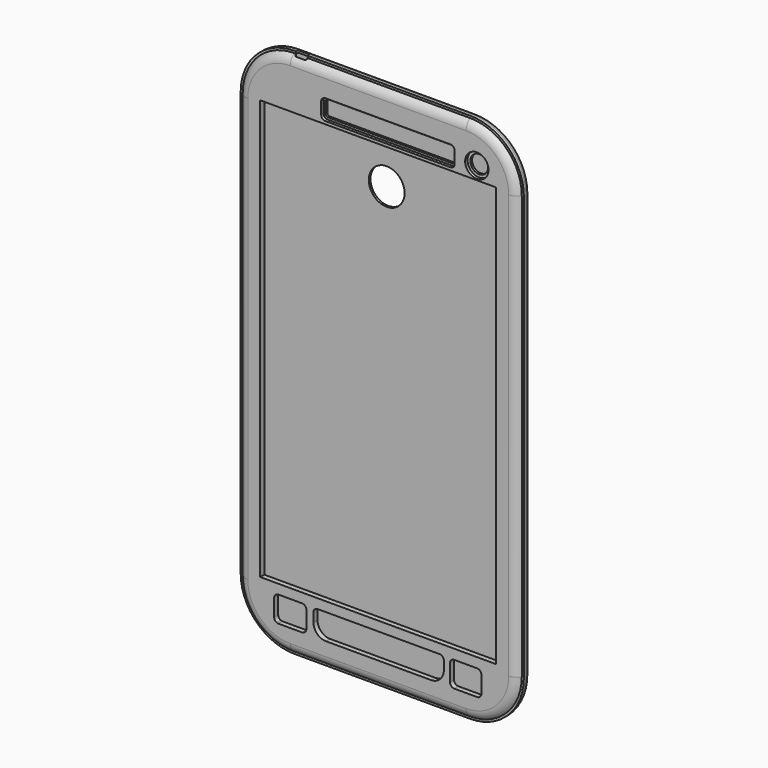
from build123d import *

# Parameters (mm, degrees)
F1_DEPTH       = 1.8
F2_T           = -0.5
F3_TEXT_SIZE   = 14.8850909021
F4_DEPTH       = 0.4
F6_DEPTH       = 1.2
F7_T1_DEPTH    = 100.1693180323
F7_T3_DEPTH    = 41.579196465
F7_T6_ANGLE    = 90
F7_T8_ANGLE    = 90
F7_T10_ANGLE   = 90
F7_T12_ANGLE   = 90
F8_R           = 1.2
F10_W          = 55.8126681519
F10_H          = 99.2564819753
F11_DEPTH      = 5.0007207319
F13_DEPTH      = 25
F14_R          = 2.7675954625
F14_R_2        = 2.0923613447
F15_DEPTH      = 0.6937347353
F16_DEPTH      = 3
F19_DEPTH      = 25
F20_R          = 4.2318258576
F21_DEPTH      = 25
F23_DEPTH      = 10
F23_DEPTH_BACK = 25


# Not quite as in the source:
# - a fillet or chamfer that OpenCascade refuses, or shapes differently, is made with other operations: its cross-section is extruded or revolved along the edge and cut away or added
# - Text() gives the source's letters only with a copy of the font that has no kerning and outlines rounded to 1/6400 em; it was checked with that copy


with BuildPart() as f1:
    # F0 (on Front) → F1 (new body)
    with BuildSketch(Plane.XZ):
        with BuildLine():
            Line((25.4936250091, 55.1304519176), (-16.085571456, 55.1304519176))
            ThreePointArc((-16.085571456, 55.1304519176), (-25.065827577, 51.4107080387), (-28.785571456, 42.4304519176))
            Line((-28.785571456, 42.4304519176), (-28.785571456, -57.7388661146))
            ThreePointArc((-28.785571456, -57.7388661146), (-25.065827577, -66.7191222357), (-16.085571456, -70.4388661146))
            Line((-16.085571456, -70.4388661146), (25.4936250091, -70.4388661146))
            ThreePointArc((25.4936250091, -70.4388661146), (34.4738811301, -66.7191222357), (38.1936250091, -57.7388661146))
            Line((38.1936250091, -57.7388661146), (38.1936250091, 42.4304519176))
            ThreePointArc((38.1936250091, 42.4304519176), (34.4738811301, 51.4107080387), (25.4936250091, 55.1304519176))
        make_face()
    extrude(amount=F1_DEPTH)

    # F2
    f2_openings = [f1.faces().sort_by_distance(p)[0] for p in [
        (4.704027, -1.8, -7.654207),
    ]]
    offset(amount=F2_T, openings=f2_openings)

    # F3 (on face) → F4 (join)
    with BuildSketch(Plane(origin=(0, 0, 0), x_dir=(-1, 0, 0), z_dir=(0, 1, 0))):
        with Locations((-21.8003056943, 37.4392606318)):
            Text('Asus', F3_TEXT_SIZE, font='Open Sans', font_style=FontStyle.BOLD, text_align=(TextAlign.LEFT, TextAlign.BOTTOM))
        with Locations((-17.9325078553, 17.195537005)):
            Text('ZEN', F3_TEXT_SIZE, font='Open Sans', font_style=FontStyle.BOLD, text_align=(TextAlign.LEFT, TextAlign.BOTTOM))
        with Locations((-6.329114338, -3.0481866218)):
            Text('5', F3_TEXT_SIZE, font='Open Sans', font_style=FontStyle.BOLD, text_align=(TextAlign.LEFT, TextAlign.BOTTOM))
    extrude(amount=F4_DEPTH)

    # F8
    f8_edges = [f1.edges().sort_by_distance(p)[0] for p in [
        (-25.065828, 0, -66.719122),
        (4.704027, 0, -70.438866),
        (34.473881, 0, -66.719122),
        (38.193625, 0, -7.654207),
        (-28.785571, 0, -7.654207),
        (-25.065828, 0, 51.410708),
        (4.704027, 0, 55.130452),
        (34.473881, 0, 51.410708),
    ]]
    fillet(f8_edges, radius=F8_R)

    # F18 (on face) → F19 (cut)
    with BuildSketch(Plane(origin=(0, 0, -70.4388661146), x_dir=(1, 0, 0), z_dir=(0, 0, -1))):
        with BuildLine():
            Line((6.5061416602, 1.2), (2.9019118929, 1.2))
            Line((2.9019118929, 1.2), (2.9019118929, 0.8308712449))
            ThreePointArc((2.9019118929, 0.8308712449), (2.9897798586, 0.6187392105), (3.2019118929, 0.5308712449))
            Line((3.2019118929, 0.5308712449), (4.7040267766, 0.5308712449))
            Line((4.7040267766, 0.5308712449), (6.2061416602, 0.5308712449))
            ThreePointArc((6.2061416602, 0.5308712449), (6.4182736945, 0.6187392105), (6.5061416602, 0.8308712449))
            Line((6.5061416602, 0.8308712449), (6.5061416602, 1.2))
        make_face()
        Polygon((6.5061416602, 1.6659845887), (4.7040267766, 1.6659845887), (2.9019118929, 1.6659845887), (2.9019118929, 1.2), (6.5061416602, 1.2), align=None)
    extrude(amount=-F19_DEPTH, mode=Mode.SUBTRACT)

    # F20 (on face) → F21 (cut)
    with BuildSketch(Plane(origin=(0, 0, 0), x_dir=(-1, 0, 0), z_dir=(0, 1, 0))):
        with Locations((-4.7040267766, 33.0976899713)):
            Circle(F20_R)
    extrude(amount=-F21_DEPTH, mode=Mode.SUBTRACT)


with BuildPart() as f6:
    # F5 (on face) → F6 (new body)
    with BuildSketch(Plane.XZ.offset(1.8)):
        with BuildLine():
            ThreePointArc((37.6936250091, 42.4304519176), (34.1203277395, 51.0571546481), (25.4936250091, 54.6304519176))
            Line((25.4936250091, 54.6304519176), (-16.085571456, 54.6304519176))
            ThreePointArc((-16.085571456, 54.6304519176), (-24.7122741864, 51.0571546481), (-28.285571456, 42.4304519176))
            Line((-28.285571456, 42.4304519176), (-28.285571456, -57.7388661146))
            ThreePointArc((-28.285571456, -57.7388661146), (-24.7122741864, -66.3655688451), (-16.085571456, -69.9388661146))
            Line((-16.085571456, -69.9388661146), (25.4936250091, -69.9388661146))
            ThreePointArc((25.4936250091, -69.9388661146), (34.1203277395, -66.3655688451), (37.6936250091, -57.7388661146))
            Line((37.6936250091, -57.7388661146), (37.6936250091, 42.4304519176))
        make_face()
    extrude(amount=F6_DEPTH)

    # F7: fillet of radius 2.5 on 2 edges, made by hand

    # F7_s2 → F7_t1 (cut)
    with BuildSketch(Plane.XY.offset(-57.7388661146)):
        with BuildLine():
            ThreePointArc((37.6936250091, -1.8), (36.78295423, -2.6794494718), (35.5582093587, -3))
            Line((35.5582093587, -3), (35.5582093587, -3.05))
            Line((35.5582093587, -3.05), (37.6936250091, -3.05))
            Line((37.6936250091, -3.05), (37.7436250091, -3))
            ThreePointArc((37.7436250091, -3), (37.7436250091, -2.4), (37.7363333221, -1.826))
            Line((37.7363333221, -1.826), (37.6936250091, -1.8))
        make_face()
        with BuildLine():
            ThreePointArc((-28.285571456, -1.8), (-27.3749006769, -2.6794494718), (-26.1501558055, -3))
            Line((-26.1501558055, -3), (-26.1501558055, -3.05))
            Line((-26.1501558055, -3.05), (-28.285571456, -3.05))
            Line((-28.285571456, -3.05), (-28.335571456, -3))
            ThreePointArc((-28.335571456, -3), (-28.335571456, -2.4), (-28.328279769, -1.826))
            Line((-28.328279769, -1.826), (-28.285571456, -1.8))
        make_face()
    extrude(amount=F7_T1_DEPTH, mode=Mode.SUBTRACT)

    # F7_s4 → F7_t3 (cut)
    with BuildSketch(Plane.YZ.offset(-16.085571456)):
        with BuildLine():
            ThreePointArc((-1.8, 54.6304519176), (-2.6794494718, 53.7197811386), (-3, 52.4950362672))
            Line((-3, 52.4950362672), (-3.05, 52.4950362672))
            Line((-3.05, 52.4950362672), (-3.05, 54.6304519176))
            Line((-3.05, 54.6304519176), (-3, 54.6804519176))
            ThreePointArc((-3, 54.6804519176), (-2.4, 54.6804519176), (-1.826, 54.6731602307))
            Line((-1.826, 54.6731602307), (-1.8, 54.6304519176))
        make_face()
        with BuildLine():
            ThreePointArc((-1.8, -69.9388661146), (-2.6794494718, -69.0281953356), (-3, -67.8034504642))
            Line((-3, -67.8034504642), (-3.05, -67.8034504642))
            Line((-3.05, -67.8034504642), (-3.05, -69.9388661146))
            Line((-3.05, -69.9388661146), (-3, -69.9888661146))
            ThreePointArc((-3, -69.9888661146), (-2.4, -69.9888661146), (-1.826, -69.9815744276))
            Line((-1.826, -69.9815744276), (-1.8, -69.9388661146))
        make_face()
    extrude(amount=F7_T3_DEPTH, mode=Mode.SUBTRACT)

    # F7_s5 → F7_t6 (revolve, cut)
    with BuildSketch(Plane.YZ.offset(25.4936250091)):
        with BuildLine():
            ThreePointArc((-1.8, -69.9388661146), (-2.6794494718, -69.0281953356), (-3, -67.8034504642))
            Line((-3, -67.8034504642), (-3.05, -67.8034504642))
            Line((-3.05, -67.8034504642), (-3.05, -69.9388661146))
            Line((-3.05, -69.9388661146), (-3, -69.9888661146))
            ThreePointArc((-3, -69.9888661146), (-2.4, -69.9888661146), (-1.826, -69.9815744276))
            Line((-1.826, -69.9815744276), (-1.8, -69.9388661146))
        make_face()
    revolve(axis=Axis((25.4936250091, -3, -57.7388661146), (0, -1, 0)), revolution_arc=F7_T6_ANGLE, mode=Mode.SUBTRACT)

    # F7_s7 → F7_t8 (revolve, cut)
    with BuildSketch(Plane.XY.offset(42.4304519176)):
        with BuildLine():
            ThreePointArc((37.6936250091, -1.8), (36.78295423, -2.6794494718), (35.5582093587, -3))
            Line((35.5582093587, -3), (35.5582093587, -3.05))
            Line((35.5582093587, -3.05), (37.6936250091, -3.05))
            Line((37.6936250091, -3.05), (37.7436250091, -3))
            ThreePointArc((37.7436250091, -3), (37.7436250091, -2.4), (37.7363333221, -1.826))
            Line((37.7363333221, -1.826), (37.6936250091, -1.8))
        make_face()
    revolve(axis=Axis((25.4936250091, -3, 42.4304519176), (0, -1, 0)), revolution_arc=F7_T8_ANGLE, mode=Mode.SUBTRACT)

    # F7_s9 → F7_t10 (revolve, cut)
    with BuildSketch(Plane.YZ.offset(-16.085571456)):
        with BuildLine():
            ThreePointArc((-1.8, 54.6304519176), (-2.6794494718, 53.7197811386), (-3, 52.4950362672))
            Line((-3, 52.4950362672), (-3.05, 52.4950362672))
            Line((-3.05, 52.4950362672), (-3.05, 54.6304519176))
            Line((-3.05, 54.6304519176), (-3, 54.6804519176))
            ThreePointArc((-3, 54.6804519176), (-2.4, 54.6804519176), (-1.826, 54.6731602307))
            Line((-1.826, 54.6731602307), (-1.8, 54.6304519176))
        make_face()
    revolve(axis=Axis((-16.085571456, -3, 42.4304519176), (0, -1, 0)), revolution_arc=F7_T10_ANGLE, mode=Mode.SUBTRACT)

    # F7_s11 → F7_t12 (revolve, cut)
    with BuildSketch(Plane.XY.offset(-57.7388661146)):
        with BuildLine():
            ThreePointArc((-28.285571456, -1.8), (-27.3749006769, -2.6794494718), (-26.1501558055, -3))
            Line((-26.1501558055, -3), (-26.1501558055, -3.05))
            Line((-26.1501558055, -3.05), (-28.285571456, -3.05))
            Line((-28.285571456, -3.05), (-28.335571456, -3))
            ThreePointArc((-28.335571456, -3), (-28.335571456, -2.4), (-28.328279769, -1.826))
            Line((-28.328279769, -1.826), (-28.285571456, -1.8))
        make_face()
    revolve(axis=Axis((-16.085571456, -3, -57.7388661146), (0, -1, 0)), revolution_arc=F7_T12_ANGLE, mode=Mode.SUBTRACT)

    # F10 (on face) → F11 (cut)
    with BuildSketch(Plane.XZ.offset(3)):
        with Locations((4.7040267766, -6.6294241697)):
            Rectangle(F10_W, F10_H)
    extrude(amount=-F11_DEPTH, mode=Mode.SUBTRACT)

    # F12 (on face) → F13 (cut)
    with BuildSketch(Plane.XZ.offset(3)):
        with BuildLine():
            ThreePointArc((-12.2817195952, -59.5123114288), (-12.574612814, -58.8052046476), (-13.2817195952, -58.5123114288))
            Line((-13.2817195952, -58.5123114288), (-18.9017766863, -58.5123114288))
            ThreePointArc((-18.9017766863, -58.5123114288), (-19.6088834675, -58.8052046476), (-19.9017766863, -59.5123114288))
            Line((-19.9017766863, -59.5123114288), (-19.9017766863, -63.5656511188))
            ThreePointArc((-19.9017766863, -63.5656511188), (-19.7562864222, -64.0850864961), (-19.3621504639, -64.453376293))
            ThreePointArc((-19.3621504639, -64.453376293), (-19.2387093732, -64.499454064), (-19.1142862352, -64.5428101087))
            ThreePointArc((-19.1142862352, -64.5428101087), (-19.0086434493, -64.559924469), (-18.9017766863, -64.5656511188))
            Line((-18.9017766863, -64.5656511188), (-13.3337015286, -64.5656511188))
            ThreePointArc((-13.3337015286, -64.5656511188), (-12.5898379698, -64.2575327441), (-12.2817195952, -63.5136691853))
            Line((-12.2817195952, -63.5136691853), (-12.2817195952, -59.5123114288))
        make_face()
        with BuildLine():
            Line((29.1073294297, -63.5656511188), (29.1073294297, -59.5850522459))
            ThreePointArc((29.1073294297, -59.5850522459), (28.8144362109, -58.8779454647), (28.1073294297, -58.5850522459))
            Line((28.1073294297, -58.5850522459), (22.6829676867, -58.5850522459))
            ThreePointArc((22.6829676867, -58.5850522459), (21.9758609055, -58.8779454647), (21.6829676867, -59.5850522459))
            Line((21.6829676867, -59.5850522459), (21.6829676867, -63.5656511188))
            ThreePointArc((21.6829676867, -63.5656511188), (21.9758609055, -64.2727578999), (22.6829676867, -64.5656511188))
            Line((22.6829676867, -64.5656511188), (28.1073294297, -64.5656511188))
            ThreePointArc((28.1073294297, -64.5656511188), (28.8144362109, -64.2727578999), (29.1073294297, -63.5656511188))
        make_face()
        with BuildLine():
            ThreePointArc((20.2198089153, -59.5123114288), (19.9269156964, -58.8052046476), (19.2198089153, -58.5123114288))
            Line((19.2198089153, -58.5123114288), (-9.6241041794, -58.5123114288))
            ThreePointArc((-9.6241041794, -58.5123114288), (-10.3312109606, -58.8052046476), (-10.6241041794, -59.5123114288))
            Line((-10.6241041794, -59.5123114288), (-10.6241041794, -61.5703942418))
            ThreePointArc((-10.6241041794, -61.5703942418), (-9.745424523, -63.6917145854), (-7.6241041794, -64.5703942418))
            Line((-7.6241041794, -64.5703942418), (17.2198089153, -64.5703942418))
            ThreePointArc((17.2198089153, -64.5703942418), (19.3411292588, -63.6917145854), (20.2198089153, -61.5703942418))
            Line((20.2198089153, -61.5703942418), (20.2198089153, -59.5123114288))
        make_face()
    extrude(amount=-F13_DEPTH, mode=Mode.SUBTRACT)

    # F14 (on face) → F15 (cut)
    with BuildSketch(Plane.XZ.offset(3)):
        with BuildLine():
            Line((21.8011573888, 48.4449677169), (-7.7840846498, 48.4449677169))
            ThreePointArc((-7.7840846498, 48.4449677169), (-8.4911914309, 48.1520744981), (-8.7840846498, 47.4449677169))
            Line((-8.7840846498, 47.4449677169), (-8.7840846498, 44.6754697382))
            ThreePointArc((-8.7840846498, 44.6754697382), (-8.4911914309, 43.9683629571), (-7.7840846498, 43.6754697382))
            Line((-7.7840846498, 43.6754697382), (21.8011573888, 43.6754697382))
            ThreePointArc((21.8011573888, 43.6754697382), (22.50826417, 43.9683629571), (22.8011573888, 44.6754697382))
            Line((22.8011573888, 44.6754697382), (22.8011573888, 47.4449677169))
            ThreePointArc((22.8011573888, 47.4449677169), (22.50826417, 48.1520744981), (21.8011573888, 48.4449677169))
        make_face()
        with BuildLine():
            Line((21.8011573888, 44.1754697382), (-7.7840846498, 44.1754697382))
            ThreePointArc((-7.7840846498, 44.1754697382), (-8.1376380403, 44.3219163477), (-8.2840846498, 44.6754697382))
            Line((-8.2840846498, 44.6754697382), (-8.2840846498, 47.4449677169))
            ThreePointArc((-8.2840846498, 47.4449677169), (-8.1376380403, 47.7985211075), (-7.7840846498, 47.9449677169))
            Line((-7.7840846498, 47.9449677169), (21.8011573888, 47.9449677169))
            ThreePointArc((21.8011573888, 47.9449677169), (22.1547107794, 47.7985211075), (22.3011573888, 47.4449677169))
            Line((22.3011573888, 47.4449677169), (22.3011573888, 44.6754697382))
            ThreePointArc((22.3011573888, 44.6754697382), (22.1547107794, 44.3219163477), (21.8011573888, 44.1754697382))
        make_face(mode=Mode.SUBTRACT)
        with BuildLine():
            ThreePointArc((-8.2840846498, 44.6754697382), (-8.1376380403, 44.3219163477), (-7.7840846498, 44.1754697382))
            Line((-7.7840846498, 44.1754697382), (21.8011573888, 44.1754697382))
            ThreePointArc((21.8011573888, 44.1754697382), (22.1547107794, 44.3219163477), (22.3011573888, 44.6754697382))
            Line((22.3011573888, 44.6754697382), (22.3011573888, 47.4449677169))
            ThreePointArc((22.3011573888, 47.4449677169), (22.1547107794, 47.7985211075), (21.8011573888, 47.9449677169))
            Line((21.8011573888, 47.9449677169), (-7.7840846498, 47.9449677169))
            ThreePointArc((-7.7840846498, 47.9449677169), (-8.1376380403, 47.7985211075), (-8.2840846498, 47.4449677169))
            Line((-8.2840846498, 47.4449677169), (-8.2840846498, 44.6754697382))
        make_face()
        with Locations((28.0271082409, 46.0602187276)):
            Circle(F14_R)
        with Locations((28.0271082409, 46.0602187276)):
            Circle(F14_R_2, mode=Mode.SUBTRACT)
        with Locations((28.0271082409, 46.0602187276)):
            Circle(F14_R_2)
    extrude(amount=-F15_DEPTH, mode=Mode.SUBTRACT)


with BuildPart() as f16:
    # F14 (on face) → F16 (new body)
    with BuildSketch(Plane.XZ.offset(3)):
        with BuildLine():
            ThreePointArc((-8.2840846498, 44.6754697382), (-8.1376380403, 44.3219163477), (-7.7840846498, 44.1754697382))
            Line((-7.7840846498, 44.1754697382), (21.8011573888, 44.1754697382))
            ThreePointArc((21.8011573888, 44.1754697382), (22.1547107794, 44.3219163477), (22.3011573888, 44.6754697382))
            Line((22.3011573888, 44.6754697382), (22.3011573888, 47.4449677169))
            ThreePointArc((22.3011573888, 47.4449677169), (22.1547107794, 47.7985211075), (21.8011573888, 47.9449677169))
            Line((21.8011573888, 47.9449677169), (-7.7840846498, 47.9449677169))
            ThreePointArc((-7.7840846498, 47.9449677169), (-8.1376380403, 47.7985211075), (-8.2840846498, 47.4449677169))
            Line((-8.2840846498, 47.4449677169), (-8.2840846498, 44.6754697382))
        make_face()
    extrude(amount=-F16_DEPTH)


with BuildPart() as f16b:
    # F14 (on face) → F16, piece 2 (new body)
    with BuildSketch(Plane.XZ.offset(3)):
        with Locations((28.0271082409, 46.0602187276)):
            Circle(F14_R_2)
    extrude(amount=-F16_DEPTH)


with BuildPart() as f6_1:
    add(f6.part)

    # F17: cut F16, F16b
    add(f16.part, mode=Mode.SUBTRACT)
    add(f16b.part, mode=Mode.SUBTRACT)


with BuildPart() as f23_tool:
    # F22 (on face) → F23 (new body, two sides)
    with BuildSketch(Plane.XY.offset(55.1304519176)) as f23_sk:
        with BuildLine():
            Line((-13.3054918553, -1.2), (-15.2593517126, -1.2))
            ThreePointArc((-15.2593517126, -1.2), (-15.5421944251, -1.3171572875), (-15.6593517126, -1.6))
            Line((-15.6593517126, -1.6), (-15.6593517126, -1.8))
            Line((-15.6593517126, -1.8), (-12.9054918553, -1.8))
            Line((-12.9054918553, -1.8), (-12.9054918553, -1.6))
            ThreePointArc((-12.9054918553, -1.6), (-13.0226491428, -1.3171572875), (-13.3054918553, -1.2))
        make_face()
        with BuildLine():
            Line((-12.9054918553, -1.8), (-15.6593517126, -1.8))
            Line((-15.6593517126, -1.8), (-15.6593517126, -1.8365227835))
            ThreePointArc((-15.6593517126, -1.8365227835), (-15.5421944251, -2.119365496), (-15.2593517126, -2.2365227835))
            Line((-15.2593517126, -2.2365227835), (-13.3054918553, -2.2365227835))
            ThreePointArc((-13.3054918553, -2.2365227835), (-13.0226491428, -2.119365496), (-12.9054918553, -1.8365227835))
            Line((-12.9054918553, -1.8365227835), (-12.9054918553, -1.8))
        make_face()
    extrude(amount=-F23_DEPTH)
    extrude(f23_sk.sketch, amount=F23_DEPTH_BACK)


with BuildPart() as f1_1:
    add(f1.part)

    # F23: cut by f23_tool
    add(f23_tool.part, mode=Mode.SUBTRACT)


with BuildPart() as f6_2:
    add(f6_1.part)

    # F23: cut by f23_tool
    add(f23_tool.part, mode=Mode.SUBTRACT)


solid = Compound([f1_1.part, f6_2.part])
